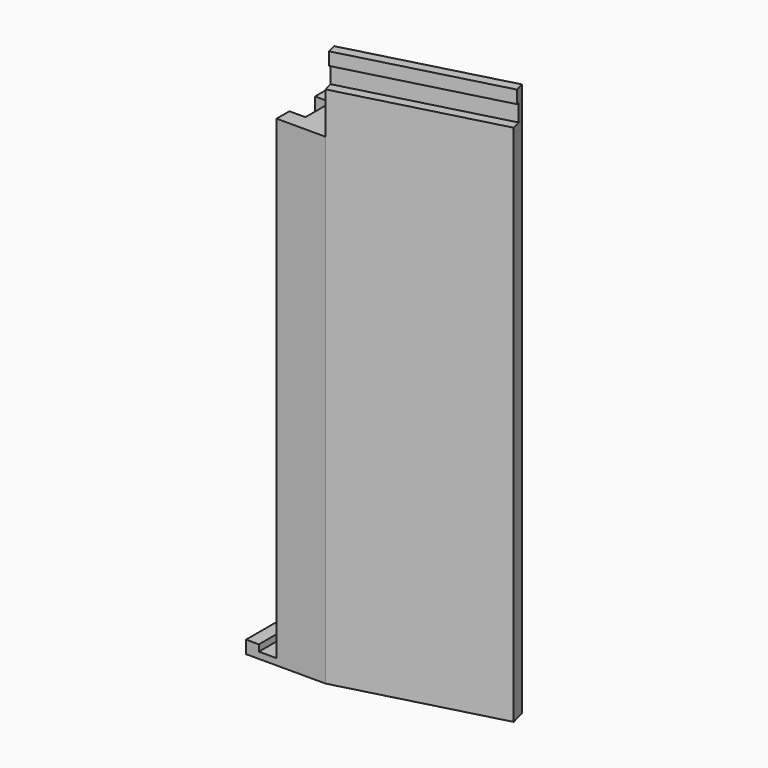
from build123d import *
from build123d import SkipClean  # not in build123d's __all__

# Parameters (mm, degrees)
F0_W      = 4
F0_H      = 20
F1_DEPTH  = 4
F2_W      = 5.5
F2_H      = 20
F3_DEPTH  = 2
F4_W      = 5
F4_H      = 20
F5_DEPTH  = 10
F6_W      = 5
F6_H      = 20
F7_DEPTH  = 150
F8_W      = 5
F8_H      = 5
F9_DEPTH  = 140
F10_W     = 5
F10_H     = 163
F11_DEPTH = 50
F12_W     = 9.4903359083
F12_H     = 16
F13_DEPTH = 20
F14_W     = 15.6903359083
F14_H     = 16
F15_DEPTH = 30
F17_DEPTH = 16
F19_DEPTH = 5.5
F21_DEPTH = 4


with BuildPart() as f1:
    # F0 (on Top) → F1 (new body)
    with BuildSketch(Plane.XY):
        with Locations((2, 10)):
            Rectangle(F0_W, F0_H)
    extrude(amount=F1_DEPTH)

    # F2 (on Top) → F3 (join)
    with BuildSketch(Plane.XY):
        with Locations((6.75, 10)):
            Rectangle(F2_W, F2_H)
    extrude(amount=F3_DEPTH)

    # F4 (on Top) → F5 (join)
    with BuildSketch(Plane.XY):
        with Locations((12, 10)):
            Rectangle(F4_W, F4_H)
    extrude(amount=F5_DEPTH)

    # F6 (on Top) → F7 (join)
    with BuildSketch(Plane.XY):
        with Locations((17, 10)):
            Rectangle(F6_W, F6_H)
        Polygon((24.8, 0), (19.5, 20), (19.5, 0), align=None)
    extrude(amount=F7_DEPTH)

    # F8 (on face) → F9 (join)
    with BuildSketch(Plane.XY.offset(10)):
        with Locations((12, 17.5)):
            Rectangle(F8_W, F8_H)
        with Locations((12, 2.5)):
            Rectangle(F8_W, F8_H)
    extrude(amount=F9_DEPTH)

    # F10 (on face) → F11 (join)
    with BuildSketch(Plane(origin=(23.17269733, 6.1407647925, 0), x_dir=(-0.2561582385, 0.9666348622, 0), z_dir=(0.9666348622, 0.2561582385, 0))):
        with Locations((-3.8527243145, 81.5)):
            Rectangle(F10_W, F10_H)
    extrude(amount=F11_DEPTH)

    # F12 (on face) → F13 (join)
    with BuildSketch(Plane(origin=(23.17269733, 6.1407647925, 0), x_dir=(-0.2561582385, 0.9666348622, 0), z_dir=(0.9666348622, 0.2561582385, 0))):
        Polygon((14.3376115938, 0), (14.3376115938, 150), (8.1376115938, 150), (8.1376115938, 16), (8.1376115938, 0), align=None)
        with Locations((3.3924436397, 8)):
            Rectangle(F12_W, F12_H)
    extrude(amount=F13_DEPTH)

    # F14 (on face) → F15 (join)
    with BuildSketch(Plane(origin=(42.5053945744, 11.2639295622, 0), x_dir=(-0.2561582385, 0.9666348622, 0), z_dir=(0.9666348622, 0.2561582385, 0))):
        with Locations((6.4924436397, 8)):
            Rectangle(F14_W, F14_H)
    extrude(amount=F15_DEPTH)

    # F16 (on face) → F17 (cut)
    with BuildSketch(Plane.XY.offset(16)):
        Polygon((67.8317431109, 32.8079119244), (38.8326972444, 25.1231647698), (71.8509519185, 17.6410862355), align=None)
    extrude(amount=-F17_DEPTH, mode=Mode.SUBTRACT)

    # F18 (on face) → F19 (join)
    with BuildSketch(Plane.XY.offset(163)):
        Polygon((71.8509519185, 17.6410862355), (23.5192088076, 4.8331743111), (24.0315252845, 2.8999045867), (72.3632683954, 15.707816511), align=None)
    extrude(amount=F19_DEPTH)

    # F20 (on face) → F21 (join)
    with BuildSketch(Plane.XY.offset(168.5)):
        Polygon((71.8509515411, 17.6410861355), (23.5192088076, 4.8331743111), (24.287683523, 1.9332697244), (72.6194262566, 14.7411815488), align=None)
    with SkipClean():  # cleaning this boolean's faces spoils the solid; the shape is the same uncleaned
        extrude(amount=F21_DEPTH)


solid = f1.part
